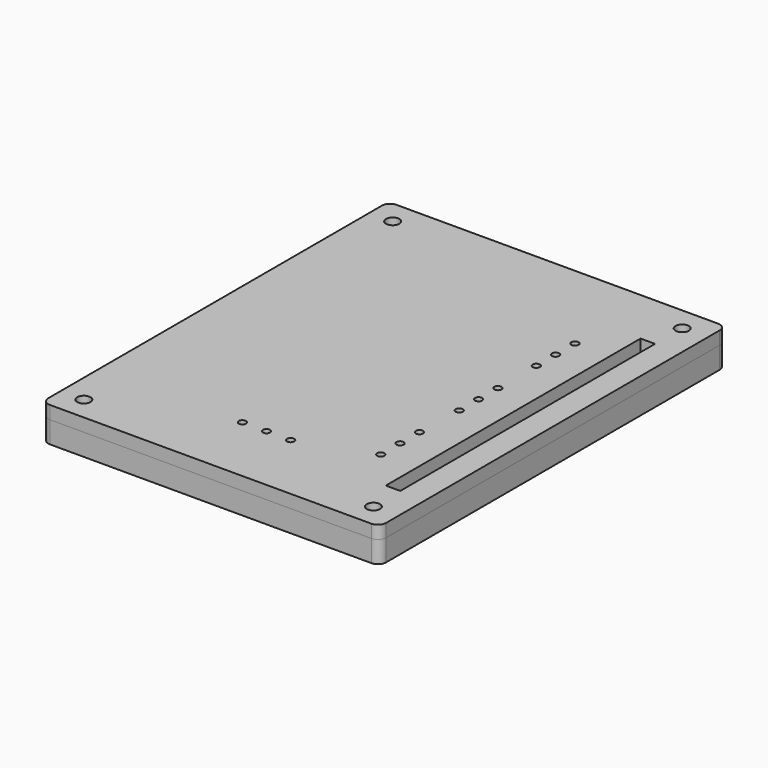
from build123d import *

# Parameters (mm, degrees)
F0_W     = 64.8
F0_H     = 85
F0_R     = 1.375
F0_W_2   = 40
F0_H_2   = 3
F0_W_3   = 15
F0_H_3   = 3.5
F0_W_4   = 3.5
F0_H_4   = 15
F0_W_5   = 3
F0_H_5   = 66
F0_R_2   = 0.75
F1_DEPTH = 2.7
F2_DEPTH = 4.5
F3_DEPTH = 0.7


# Not quite as in the source:
# - a feature names something its author has since deleted; it is built from what else it names


with BuildPart() as f1:
    # F0 (on Top) → F1 (new body)
    with BuildSketch(Plane.XY):
        with BuildLine():
            Line((33.489, 44.9169387996), (-33.111, 44.9169387996))
            ThreePointArc((-33.111, 44.9169387996), (-34.313081528, 44.4190203276), (-34.811, 43.2169387996))
            Line((-34.811, 43.2169387996), (-34.811, -43.1830612004))
            ThreePointArc((-34.811, -43.1830612004), (-34.313081528, -44.3851427284), (-33.111, -44.8830612004))
            Line((-33.111, -44.8830612004), (33.489, -44.8830612004))
            ThreePointArc((33.489, -44.8830612004), (34.691081528, -44.3851427284), (35.189, -43.1830612004))
            Line((35.189, -43.1830612004), (35.189, 43.2169387996))
            ThreePointArc((35.189, 43.2169387996), (34.691081528, 44.4190203276), (33.489, 44.9169387996))
        make_face()
        with Locations((-0.377, 0.6012101471)):
            Rectangle(F0_W, F0_H, mode=Mode.SUBTRACT)
        with Locations((-0.377, 0.6012101471)):
            Rectangle(F0_W, F0_H)
        with Locations((-30.0036408007, -39.9986840785)):
            Circle(F0_R, mode=Mode.SUBTRACT)
        with Locations((0, -37.9998721182)):
            Rectangle(F0_W_2, F0_H_2, mode=Mode.SUBTRACT)
        with Locations((0, -30.1813874394)):
            Rectangle(F0_W_3, F0_H_3, mode=Mode.SUBTRACT)
        with Locations((30.0036408007, -39.9986840785)):
            Circle(F0_R, mode=Mode.SUBTRACT)
        with Locations((19.5379477396, -19.9982114275)):
            Rectangle(F0_W_4, F0_H_4, mode=Mode.SUBTRACT)
        with Locations((19.8054168016, 0)):
            Rectangle(F0_W_4, F0_H_4, mode=Mode.SUBTRACT)
        with Locations((28.473, 0)):
            Rectangle(F0_W_5, F0_H_5, mode=Mode.SUBTRACT)
        with Locations((-30.0036408007, 39.9986840785)):
            Circle(F0_R, mode=Mode.SUBTRACT)
        with Locations((19.773574583, 19.9999746518)):
            Rectangle(F0_W_4, F0_H_4, mode=Mode.SUBTRACT)
        with Locations((30.0036408007, 39.9986840785)):
            Circle(F0_R, mode=Mode.SUBTRACT)
        with Locations((0, -37.9998721182)):
            Rectangle(F0_W_2, F0_H_2)
        with Locations((19.8054168016, 0)):
            Rectangle(F0_W_4, F0_H_4)
        with Locations((19.8054168016, -5)):
            Circle(F0_R_2, mode=Mode.SUBTRACT)
        with Locations((19.8054168016, 0)):
            Circle(F0_R_2, mode=Mode.SUBTRACT)
        with Locations((19.8054168016, 5)):
            Circle(F0_R_2, mode=Mode.SUBTRACT)
        with Locations((19.773574583, 19.9999746518)):
            Rectangle(F0_W_4, F0_H_4)
        with Locations((19.773574583, 14.9999746518)):
            Circle(F0_R_2, mode=Mode.SUBTRACT)
        with Locations((19.773574583, 19.9999746518)):
            Circle(F0_R_2, mode=Mode.SUBTRACT)
        with Locations((19.773574583, 24.9999746518)):
            Circle(F0_R_2, mode=Mode.SUBTRACT)
        with Locations((19.5379477396, -19.9982114275)):
            Rectangle(F0_W_4, F0_H_4)
        with Locations((19.5379477396, -24.9982114275)):
            Circle(F0_R_2, mode=Mode.SUBTRACT)
        with Locations((19.5379477396, -19.9982114275)):
            Circle(F0_R_2, mode=Mode.SUBTRACT)
        with Locations((19.5379477396, -14.9982114275)):
            Circle(F0_R_2, mode=Mode.SUBTRACT)
        with Locations((0, -30.1813874394)):
            Rectangle(F0_W_3, F0_H_3)
        with Locations((-5, -30.1813874394)):
            Circle(F0_R_2, mode=Mode.SUBTRACT)
        with Locations((0, -30.1813874394)):
            Circle(F0_R_2, mode=Mode.SUBTRACT)
        with Locations((5, -30.1813874394)):
            Circle(F0_R_2, mode=Mode.SUBTRACT)
    extrude(amount=F1_DEPTH)

    # F0 (on Top) → F3 (cut)
    with BuildSketch(Plane.XY):
        with Locations((0, -30.1813874394)):
            Rectangle(F0_W_3, F0_H_3)
        with Locations((-5, -30.1813874394)):
            Circle(F0_R_2, mode=Mode.SUBTRACT)
        with Locations((0, -30.1813874394)):
            Circle(F0_R_2, mode=Mode.SUBTRACT)
        with Locations((5, -30.1813874394)):
            Circle(F0_R_2, mode=Mode.SUBTRACT)
        with Locations((19.5379477396, -19.9982114275)):
            Rectangle(F0_W_4, F0_H_4)
        with Locations((19.5379477396, -24.9982114275)):
            Circle(F0_R_2, mode=Mode.SUBTRACT)
        with Locations((19.5379477396, -19.9982114275)):
            Circle(F0_R_2, mode=Mode.SUBTRACT)
        with Locations((19.5379477396, -14.9982114275)):
            Circle(F0_R_2, mode=Mode.SUBTRACT)
        with Locations((19.8054168016, 0)):
            Rectangle(F0_W_4, F0_H_4)
        with Locations((19.8054168016, -5)):
            Circle(F0_R_2, mode=Mode.SUBTRACT)
        with Locations((19.8054168016, 0)):
            Circle(F0_R_2, mode=Mode.SUBTRACT)
        with Locations((19.8054168016, 5)):
            Circle(F0_R_2, mode=Mode.SUBTRACT)
        with Locations((19.773574583, 19.9999746518)):
            Rectangle(F0_W_4, F0_H_4)
        with Locations((19.773574583, 14.9999746518)):
            Circle(F0_R_2, mode=Mode.SUBTRACT)
        with Locations((19.773574583, 19.9999746518)):
            Circle(F0_R_2, mode=Mode.SUBTRACT)
        with Locations((19.773574583, 24.9999746518)):
            Circle(F0_R_2, mode=Mode.SUBTRACT)
        with Locations((5, -30.1813874394)):
            Circle(F0_R_2)
        with Locations((19.8054168016, 5)):
            Circle(F0_R_2)
        with Locations((19.8054168016, -5)):
            Circle(F0_R_2)
        with Locations((19.773574583, 14.9999746518)):
            Circle(F0_R_2)
        with Locations((19.773574583, 24.9999746518)):
            Circle(F0_R_2)
        with Locations((19.5379477396, -24.9982114275)):
            Circle(F0_R_2)
        with Locations((19.5379477396, -14.9982114275)):
            Circle(F0_R_2)
        with Locations((19.773574583, 19.9999746518)):
            Circle(F0_R_2)
        with Locations((-5, -30.1813874394)):
            Circle(F0_R_2)
        with Locations((0, -30.1813874394)):
            Circle(F0_R_2)
        with Locations((19.5379477396, -19.9982114275)):
            Circle(F0_R_2)
        with Locations((19.8054168016, 0)):
            Circle(F0_R_2)
    extrude(amount=F3_DEPTH, mode=Mode.SUBTRACT)


with BuildPart() as f2:
    # F0 (on Top) → F2 (new body)
    with BuildSketch(Plane.XY):
        with BuildLine():
            Line((33.489, 44.9169387996), (-33.111, 44.9169387996))
            ThreePointArc((-33.111, 44.9169387996), (-34.313081528, 44.4190203276), (-34.811, 43.2169387996))
            Line((-34.811, 43.2169387996), (-34.811, -43.1830612004))
            ThreePointArc((-34.811, -43.1830612004), (-34.313081528, -44.3851427284), (-33.111, -44.8830612004))
            Line((-33.111, -44.8830612004), (33.489, -44.8830612004))
            ThreePointArc((33.489, -44.8830612004), (34.691081528, -44.3851427284), (35.189, -43.1830612004))
            Line((35.189, -43.1830612004), (35.189, 43.2169387996))
            ThreePointArc((35.189, 43.2169387996), (34.691081528, 44.4190203276), (33.489, 44.9169387996))
        make_face()
        with Locations((-0.377, 0.6012101471)):
            Rectangle(F0_W, F0_H, mode=Mode.SUBTRACT)
    extrude(amount=-F2_DEPTH)


with BuildPart() as f2b:
    # F0 (on Top) → F2, piece 2 (new body)
    with BuildSketch(Plane.XY):
        with Locations((0, -37.9998721182)):
            Rectangle(F0_W_2, F0_H_2)
    extrude(amount=-F2_DEPTH)


solid = Compound([f1.part, f2.part, f2b.part])
